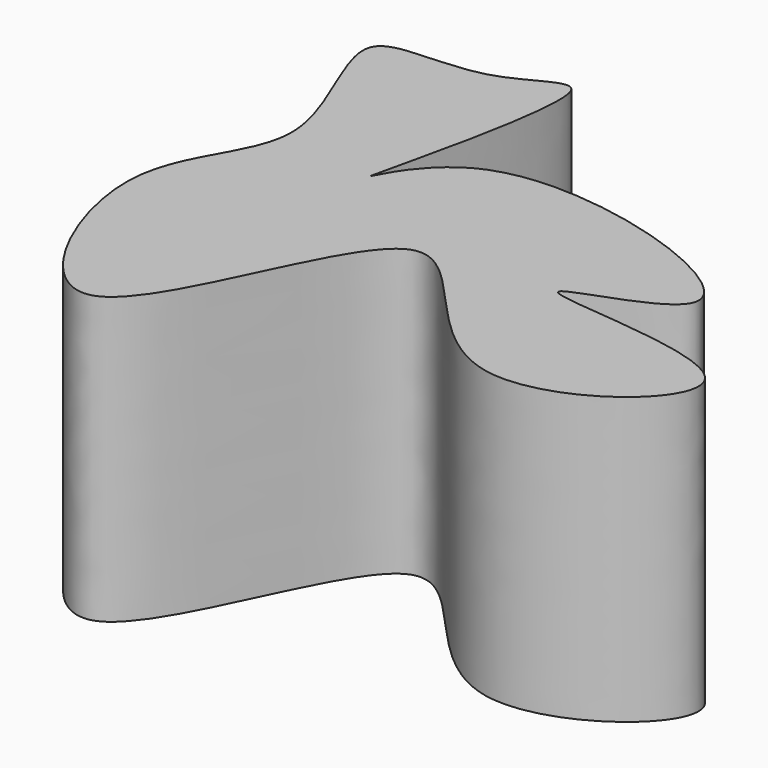
from build123d import *

# Parameters (mm, degrees)
F3_DEPTH = 25.4


# Not quite as in the source:
# - the program builds the solid bodies; features that only make, move or delete a surface that nothing else refers to are left out


with BuildPart() as f3:
    # F2 (on Top) → F3 (new body)
    with BuildSketch(Plane.XY):
        with BuildLine():
            add(Edge.make_bspline(
                [(25.7174987346, 28.3708944917), (33.479293236, 31.5269498912), (61.1414714268, 21.9665068644), (30.7037671855, 15.8377246942), (68.0178153105, 16.9797684407), (41.6380622688, -3.820621335), (28.2560453865, 29.1427953307), (17.5541510214, -16.3573177099), (2.8079813543, 14.3413943563), (15.9955590589, 22.664904938), (3.2161700265, 40.8445582271), (17.069587182, 37.6642827557), (26.217573396, 46.8113956898), (17.7173042764, 14.4790405592), (21.2649726487, 26.5604344244), (25.7174987346, 28.3708944917)],
                knots=[0, 0, 0, 0, 0.1002331682, 0.1628826278, 0.2452467611, 0.3238813165, 0.4121078489, 0.5095474981, 0.5945061426, 0.6684338122, 0.7434747527, 0.8047091928, 0.8548257792, 0.942501596, 1, 1, 1, 1], degree=3))
        make_face()
    extrude(amount=F3_DEPTH)


solid = f3.part
